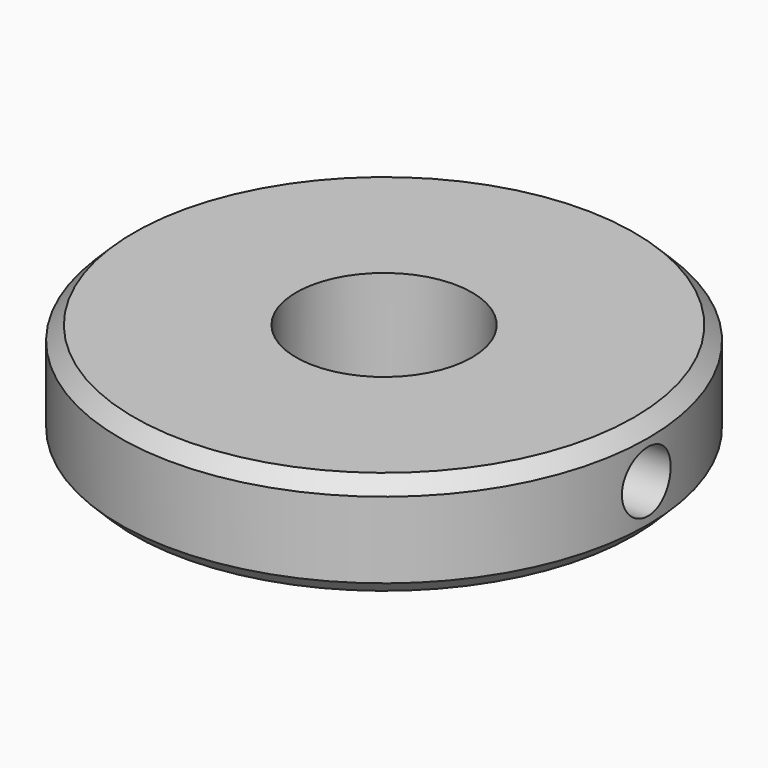
from build123d import *

# Parameters (mm, degrees)
F0_R     = 38.1
F0_R_2   = 12.7
F1_DEPTH = 15
F2_SIZE  = 2
F5_D     = 8.8
F5_DEPTH = 38.1
F5_TIP   = 2.6437867237


# Not quite as in the source:
# - a length typed as a fraction of an inch, garbled in the dataset ("3 / 203.2 mm" for 3/8 in), is restored


with BuildPart() as f1:
    # F0 (on Top) → F1 (new body)
    with BuildSketch(Plane.XY):
        Circle(F0_R)
        Circle(F0_R_2, mode=Mode.SUBTRACT)
    extrude(amount=F1_DEPTH)

    # F2
    f2_edges = [f1.edges().sort_by_distance(p)[0] for p in [
        (-38.1, 0, 15),
        (-38.1, 0, 0),
    ]]
    chamfer(f2_edges, length=F2_SIZE)

    # F5
    with Locations(Plane.YZ.offset(38.1)):
        with Locations((0, 7.5)):
            Hole(F5_D / 2, depth=F5_DEPTH)
            with Locations((0, 0, -(F5_DEPTH + F5_TIP / 2))):  # 118° drill point
                Cone(0, F5_D / 2, F5_TIP, mode=Mode.SUBTRACT)


solid = f1.part
